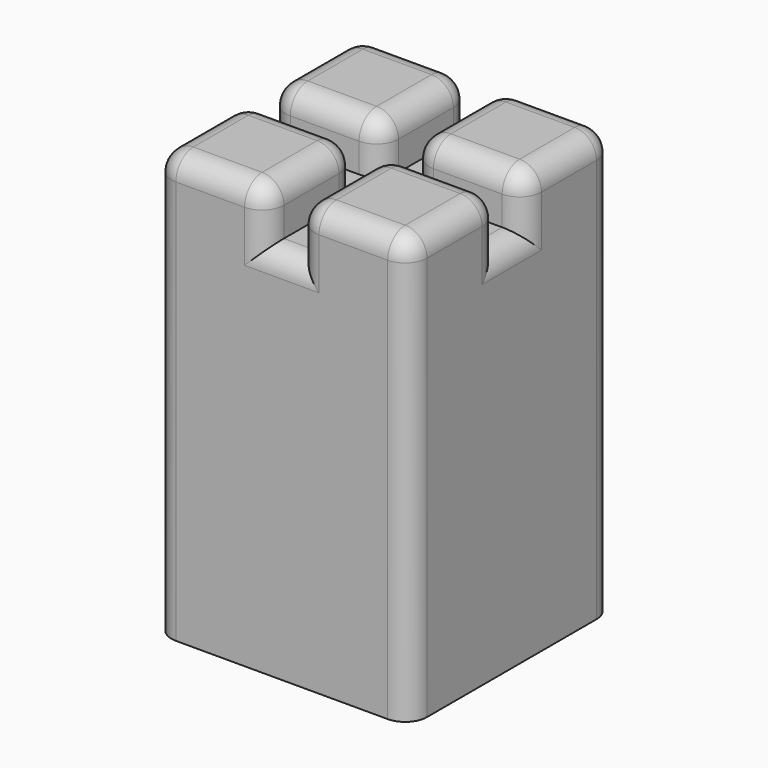
from build123d import *

# Parameters (mm, degrees)
F0_W     = 38.1
F0_H     = 38.1
F2_DEPTH = 31.75
F4_W     = 4.572
F4_H     = 16.764
F3_W     = 16.764
F3_H     = 4.572
F3_W_2   = 4.572
F3_H_2   = 16.764
F5_DEPTH = 7.62
F6_R     = 3.2591265624


with BuildPart() as f2:
    # F0 (on Top) → F2 (new body, symmetric)
    with BuildSketch(Plane.XY):
        Rectangle(F0_W, F0_H)
    extrude(amount=F2_DEPTH, both=True)

    # F4 (on face) + F3 (on face) → F5 (cut)
    with BuildSketch(Plane.XY.offset(31.75)):
        with Locations((0, 10.668)):
            Rectangle(F4_W, F4_H)
    with BuildSketch(Plane.XY.offset(31.75)):
        with Locations((-10.668, 0)):
            Rectangle(F3_W, F3_H)
        Rectangle(F3_W_2, F3_H)
        with Locations((10.668, 0)):
            Rectangle(F3_W, F3_H)
        with Locations((0, -10.668)):
            Rectangle(F3_W_2, F3_H_2)
    extrude(amount=-F5_DEPTH, mode=Mode.SUBTRACT)

    # F6
    f6_edges = [f2.edges().sort_by_distance(p)[0] for p in [
        (10.668, 19.05, 31.75),
        (19.05, 10.668, 31.75),
        (19.05, 19.05, 0),
        (2.286, -10.668, 31.75),
        (10.668, 2.286, 31.75),
        (19.05, 0, 24.13),
        (19.05, 2.286, 27.94),
        (19.05, -2.286, 27.94),
        (19.05, -10.668, 31.75),
        (19.05, -19.05, 0),
        (10.668, -19.05, 31.75),
        (2.286, -19.05, 27.94),
        (0, -19.05, 24.13),
        (-2.286, -19.05, 27.94),
        (10.668, -2.286, 31.75),
        (-19.05, -10.668, 31.75),
        (-10.668, -2.286, 31.75),
        (-2.286, -10.668, 31.75),
        (-10.668, -19.05, 31.75),
        (-19.05, -2.286, 27.94),
        (-19.05, 0, 24.13),
        (-19.05, 2.286, 27.94),
        (-19.05, 10.668, 31.75),
        (-19.05, 19.05, 0),
        (-10.668, 19.05, 31.75),
        (-10.668, 2.286, 31.75),
        (-2.286, 19.05, 27.94),
        (2.286, 19.05, 27.94),
        (0, 19.05, 24.13),
        (-2.286, 2.286, 27.94),
        (-2.286, -2.286, 27.94),
        (2.286, 2.286, 27.94),
        (2.286, -2.286, 27.94),
        (-19.05, -19.05, 0),
        (-2.286, 10.668, 31.75),
        (2.286, 10.668, 31.75),
    ]]
    fillet(f6_edges, radius=F6_R)


solid = f2.part
